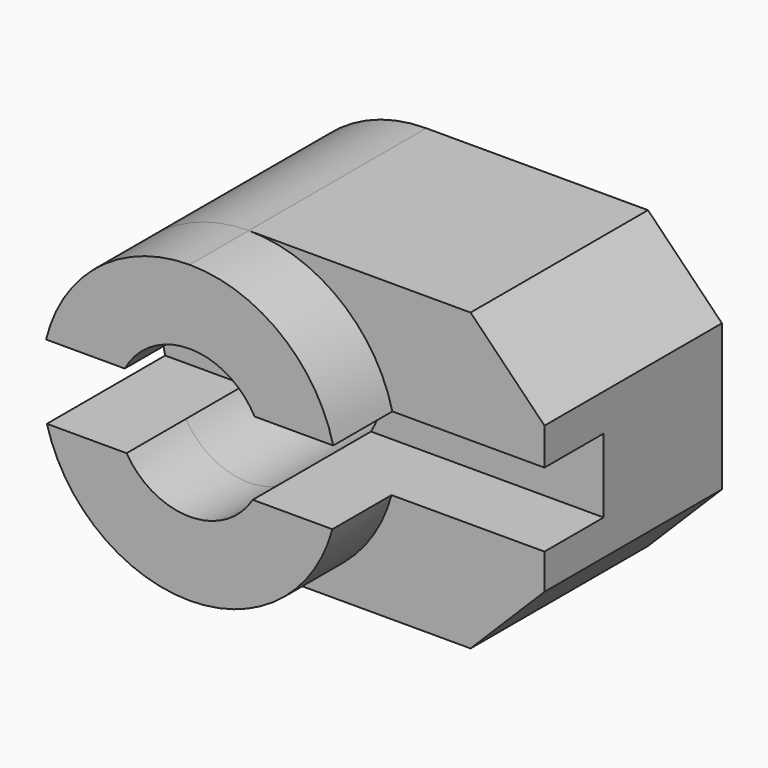
from build123d import *
from build123d import SkipClean  # not in build123d's __all__

# Parameters (mm, degrees)
F0_W     = 30
F0_H     = 15
F1_DEPTH = 20
F3_DEPTH = 15.001
F2_R     = 5
F4_DEPTH = 15.001
F5_DEPTH = 5
F6_W     = 10
F6_H     = 5
F7_DEPTH = 30.001
F9_DEPTH = 15.001


with BuildPart() as f1:
    # F0 (on Top) → F1 (new body)
    with BuildSketch(Plane.XY):
        with Locations((15, 12.5)):
            Rectangle(F0_W, F0_H)
    extrude(amount=F1_DEPTH)

    # F2 (on face) → F3 (cut, through all)
    with BuildSketch(Plane.XZ.offset(-5)):
        Polygon((30, 14.8924803361), (30, 20), (25, 20), align=None)
        Polygon((30, 0), (30, 5), (25, 0), align=None)
    extrude(amount=-F3_DEPTH, mode=Mode.SUBTRACT)

    # F2 (on face) → F4 (cut, through all)
    with BuildSketch(Plane.XZ.offset(-5)):
        with Locations((10, 10)):
            Circle(F2_R)
    extrude(amount=-F4_DEPTH, mode=Mode.SUBTRACT)

    # F2 (on face) → F5 (join)
    with BuildSketch(Plane.XZ.offset(-5)):
        with BuildLine():
            ThreePointArc((20, 10), (17.0710678119, 17.0710678119), (10, 20))
            ThreePointArc((10, 20), (2.9289321881, 17.0710678119), (0, 10))
            ThreePointArc((0, 10), (2.9289321881, 2.9289321881), (10, 0))
            ThreePointArc((10, 0), (17.0710678119, 2.9289321881), (20, 10))
        make_face()
        with Locations((10, 10)):
            Circle(F2_R, mode=Mode.SUBTRACT)
    extrude(amount=F5_DEPTH)

    # F6 (on face) → F7 (cut, through all)
    with BuildSketch(Plane.YZ.offset(30)):
        with Locations((5, 9.8924803361)):
            Rectangle(F6_W, F6_H)
    extrude(amount=-F7_DEPTH, mode=Mode.SUBTRACT)

    # F8 (on face) → F9 (cut, through all)
    with BuildSketch(Plane.XZ.offset(-5)):
        with BuildLine():
            Line((0, 20), (0, 10))
            ThreePointArc((0, 10), (2.9289321881, 17.0710678119), (10, 20))
            Line((10, 20), (0, 20))
        make_face()
        with BuildLine():
            Line((0, 10), (0, 0))
            Line((0, 0), (10, 0))
            ThreePointArc((10, 0), (2.9289321881, 2.9289321881), (0, 10))
        make_face()
    with SkipClean():  # cleaning this boolean's faces spoils the solid; the shape is the same uncleaned
        extrude(amount=-F9_DEPTH, mode=Mode.SUBTRACT)


solid = f1.part
